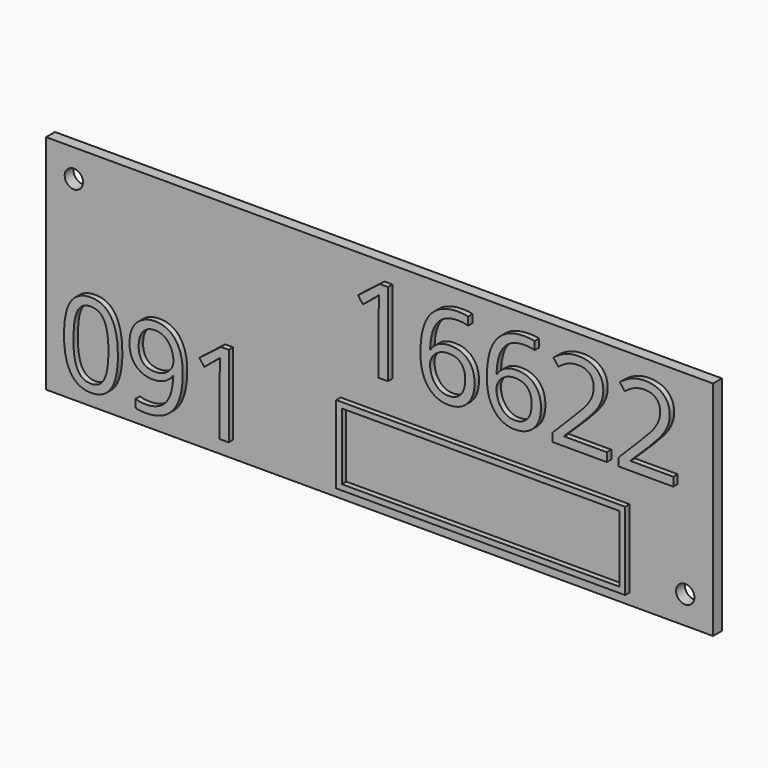
from build123d import *

# Parameters (mm, degrees)
F0_W         = 120
F0_H         = 40
F1_DEPTH     = 2
F3_D         = 3.3
F4_TEXT_SIZE = 20.9070615778
F5_DEPTH     = 1
F6_TEXT_SIZE = 20.5478077656
F7_DEPTH     = 1
F8_W         = 52
F8_H         = 14
F8_W_2       = 49.99999962
F8_H_2       = 11.99999962
F9_DEPTH     = 1


# Not quite as in the source:
# - Text() gives the source's letters only with a copy of the font that has no kerning and outlines rounded to 1/6400 em; it was checked with that copy


with BuildPart() as f1:
    # F0 (on Front) → F1 (new body)
    with BuildSketch(Plane.XZ):
        Rectangle(F0_W, F0_H)
    extrude(amount=F1_DEPTH)

    # F3 (through all)
    with Locations(Plane.XZ.offset(2)):
        with Locations((-55, 15), (55, -15)):
            Hole(F3_D / 2)

    # F4 (on face) → F5 (join)
    with BuildSketch(Plane.XZ.offset(2)):
        with Locations((-5, 2)):
            Text('16622', F4_TEXT_SIZE, font='Open Sans', text_align=(TextAlign.LEFT, TextAlign.BOTTOM))
    extrude(amount=F5_DEPTH)

    # F6 (on face) → F7 (join)
    with BuildSketch(Plane.XZ.offset(2)):
        with Locations((-57, -17)):
            Text('091', F6_TEXT_SIZE, font='Open Sans', text_align=(TextAlign.LEFT, TextAlign.BOTTOM))
    extrude(amount=F7_DEPTH)

    # F8 (on face) → F9 (join)
    with BuildSketch(Plane.XZ.offset(2)):
        with Locations((19, -11)):
            Rectangle(F8_W, F8_H)
        with Locations((19, -11)):
            Rectangle(F8_W_2, F8_H_2, mode=Mode.SUBTRACT)
    extrude(amount=F9_DEPTH)


solid = f1.part
